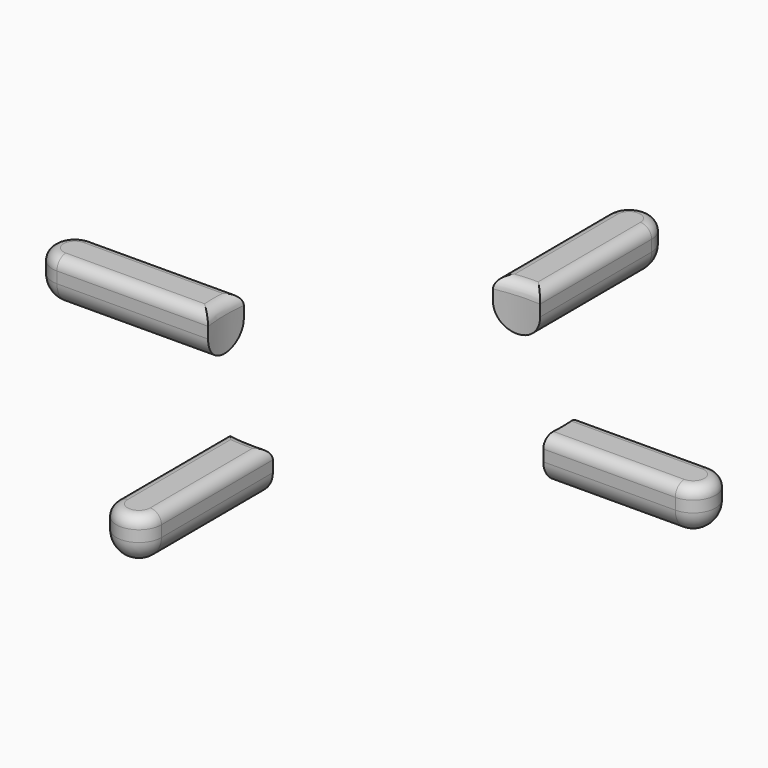
from build123d import *

# Parameters (mm, degrees)
F1_DEPTH = 4
F2_R     = 1.9999
F2_2_R   = 1.9999
F2_3_R   = 1.9999
F2_4_R   = 1.9999
F3_R     = 1
F3_2_R   = 1
F3_3_R   = 1
F3_4_R   = 1


# Not quite as in the source:
# - a fillet or chamfer is up to 0.001 mm smaller than in the source, because OpenCascade refuses the exact size


with BuildPart() as f1:
    # F0 (on Top) → F1 (new body)
    with BuildSketch(Plane.XY):
        with BuildLine():
            ThreePointArc((-2.065538543, 14.7146584401), (-0.0743129661, 14.9717221589), (1.9334062251, 14.960555095))
            Line((1.9334062251, 14.960555095), (1.8778587128, 27.4358095681))
            ThreePointArc((1.8778587128, 27.4358095681), (-0.1310266046, 29.4268845997), (-2.1221016363, 27.4179992823))
            Line((-2.1221016363, 27.4179992823), (-2.065538543, 14.7146584401))
        make_face()
    extrude(amount=F1_DEPTH)

    # F2#3 (radius 2 in the source; OpenCascade refuses exactly that, so slightly less here)
    f2_3_edges = [f1.edges().sort_by_distance(p)[0] for p in [
        (1.905632, 21.198182, 0),
    ]]
    fillet(f2_3_edges, radius=F2_3_R)

    # F3#3
    f3_3_edges = [f1.edges().sort_by_distance(p)[0] for p in [
        (-2.09382, 21.066329, 4),
        (-0.074313, 14.971722, 4),
        (1.905632, 21.198182, 4),
        (-0.131027, 29.426885, 4),
    ]]
    fillet(f3_3_edges, radius=F3_3_R)


with BuildPart() as f1b:
    # F0 (on Top) → F1, piece 2 (new body)
    with BuildSketch(Plane.XY):
        with BuildLine():
            ThreePointArc((15.7027960238, 2.0699383398), (15.8461378969, 0.0705907094), (15.7216202135, -1.9300174947))
            Line((15.7216202135, -1.9300174947), (27.4358095681, -1.8778587128))
            ThreePointArc((27.4358095681, -1.8778587128), (29.4268845997, 0.1310266046), (27.4179992823, 2.1221016363))
            Line((27.4179992823, 2.1221016363), (15.7027960238, 2.0699383398))
        make_face()
    extrude(amount=F1_DEPTH)

    # F2#2 (radius 2 in the source; OpenCascade refuses exactly that, so slightly less here)
    f2_2_edges = [f1b.edges().sort_by_distance(p)[0] for p in [
        (21.578715, -1.903938, 0),
    ]]
    fillet(f2_2_edges, radius=F2_2_R)

    # F3#2
    f3_2_edges = [f1b.edges().sort_by_distance(p)[0] for p in [
        (21.578715, -1.903938, 4),
    ]]
    fillet(f3_2_edges, radius=F3_2_R)


with BuildPart() as f1c:
    # F0 (on Top) → F1, piece 3 (new body)
    with BuildSketch(Plane.XY):
        with BuildLine():
            Line((-14.0280318673, 1.9375583925), (-27.4358095681, 1.8778587127))
            ThreePointArc((-27.4358095681, 1.8778587128), (-29.4268845997, -0.1310266046), (-27.4179992823, -2.1221016363))
            Line((-27.4179992823, -2.1221016363), (-14.0112354856, -2.062406471))
            ThreePointArc((-14.0112354856, -2.062406471), (-14.153563757, -0.0629864294), (-14.0280318673, 1.9375583925))
        make_face()
    extrude(amount=F1_DEPTH)

    # F2#4 (radius 2 in the source; OpenCascade refuses exactly that, so slightly less here)
    f2_4_edges = [f1c.edges().sort_by_distance(p)[0] for p in [
        (-20.714617, -2.092254, 0),
    ]]
    fillet(f2_4_edges, radius=F2_4_R)

    # F3#4
    f3_4_edges = [f1c.edges().sort_by_distance(p)[0] for p in [
        (-20.714617, -2.092254, 4),
        (-14.153564, -0.062986, 4),
        (-20.731921, 1.907709, 4),
        (-29.426885, -0.131027, 4),
    ]]
    fillet(f3_4_edges, radius=F3_4_R)


with BuildPart() as f1d:
    # F0 (on Top) → F1, piece 4 (new body)
    with BuildSketch(Plane.XY):
        with BuildLine():
            ThreePointArc((-1.8778587128, -27.4358095681), (0.1310266046, -29.4268845997), (2.1221016363, -27.4179992823))
            Line((2.1221016363, -27.4179992823), (2.0665876805, -14.9502811926))
            ThreePointArc((2.0665876805, -14.9502811926), (0.0590475403, -14.9793266627), (-1.9343882494, -14.7400051091))
            Line((-1.9343882494, -14.7400051091), (-1.8778587128, -27.4358095681))
        make_face()
    extrude(amount=F1_DEPTH)

    # F2 (radius 2 in the source; OpenCascade refuses exactly that, so slightly less here)
    f2_edges = [f1d.edges().sort_by_distance(p)[0] for p in [
        (2.094345, -21.18414, 0),
    ]]
    fillet(f2_edges, radius=F2_R)

    # F3
    f3_edges = [f1d.edges().sort_by_distance(p)[0] for p in [
        (-1.906123, -21.087907, 4),
        (0.131027, -29.426885, 4),
        (2.094345, -21.18414, 4),
        (0.059048, -14.979327, 4),
    ]]
    fillet(f3_edges, radius=F3_R)


solid = Compound([f1.part, f1b.part, f1c.part, f1d.part])
